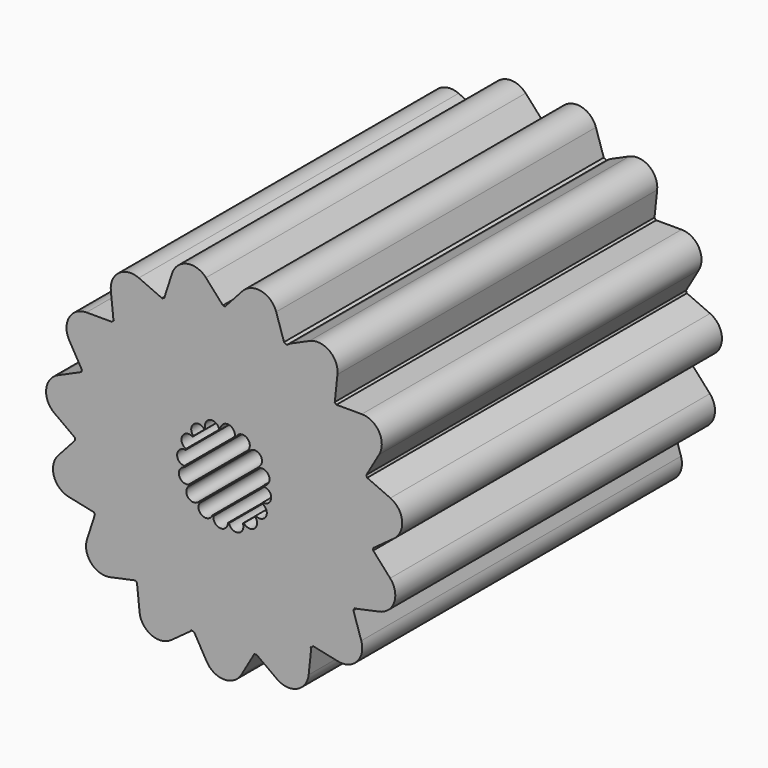
from build123d import *

# Parameters (mm, degrees)
F1_DEPTH    = 20
F2_T1_DEPTH = 28.6602540378
F2_T3_DEPTH = 21.427255965


# Not quite as in the source:
# - a fillet or chamfer that OpenCascade refuses, or shapes differently, is made with other operations: its cross-section is extruded or revolved along the edge and cut away or added


with BuildPart() as f1:
    # F0 (on Front) → F1 (new body)
    with BuildSketch(Plane.XZ):
        with BuildLine():
            Line((-32.6482919076, 40.6639489743), (-32.6758804008, 40.6333088485))
            ThreePointArc((-32.6758804008, 40.6333088485), (-33.545543461, 39.4533888073), (-34.6280952335, 38.4651546236))
            Line((-34.6280952335, 38.4651546236), (-34.6556837267, 38.4345144978))
            Line((-34.6556837267, 38.4345144978), (-31.7212409245, 37.8107794254))
            Line((-31.7212409245, 37.8107794254), (-32.6482919076, 40.6639489743))
        make_face()
        with BuildLine():
            Line((-37.6191296521, 37.1151033645), (-37.6603600082, 37.1151033645))
            ThreePointArc((-37.6603600082, 37.1151033645), (-39.1191296521, 36.971868355), (-40.5778992961, 37.1151033645))
            Line((-40.5778992961, 37.1151033645), (-40.6191296521, 37.1151033645))
            Line((-40.6191296521, 37.1151033645), (-39.1191296521, 34.5170271531))
            Line((-39.1191296521, 34.5170271531), (-37.6191296521, 37.1151033645))
        make_face()
        with BuildLine():
            Line((-40.7410773618, 37.1410241503), (-40.7787431663, 37.157794047))
            ThreePointArc((-40.7787431663, 37.157794047), (-42.1696544752, 37.6202774227), (-43.4440479302, 38.3444641829))
            Line((-43.4440479302, 38.3444641829), (-43.4817137347, 38.3612340796))
            Line((-43.4817137347, 38.3612340796), (-43.1681283449, 35.3776683935))
            Line((-43.1681283449, 35.3776683935), (-40.7410773618, 37.1410241503))
        make_face()
        with BuildLine():
            Line((-34.7565455695, 38.3612340796), (-34.794211374, 38.3444641829))
            ThreePointArc((-34.794211374, 38.3444641829), (-36.0686048291, 37.6202774227), (-37.4595161379, 37.157794047))
            Line((-37.4595161379, 37.157794047), (-37.4971819424, 37.1410241503))
            Line((-37.4971819424, 37.1410241503), (-35.0701309593, 35.3776683935))
            Line((-35.0701309593, 35.3776683935), (-34.7565455695, 38.3612340796))
        make_face()
        with BuildLine():
            Line((-43.5825755776, 38.4345144978), (-43.6101640707, 38.4651546236))
            ThreePointArc((-43.6101640707, 38.4651546236), (-44.6927158432, 39.4533888073), (-45.5623789035, 40.6333088485))
            Line((-45.5623789035, 40.6333088485), (-45.5899673966, 40.6639489743))
            Line((-45.5899673966, 40.6639489743), (-46.5170183798, 37.8107794254))
            Line((-46.5170183798, 37.8107794254), (-43.5825755776, 38.4345144978))
        make_face()
        with BuildLine():
            Line((-45.6523034437, 40.7719181749), (-45.6650443244, 40.8111305737))
            ThreePointArc((-45.6650443244, 40.8111305737), (-46.2520535243, 42.1542408972), (-46.5666135461, 43.5858753249))
            Line((-46.5666135461, 43.5858753249), (-46.5793544268, 43.6250877237))
            Line((-46.5793544268, 43.6250877237), (-48.5867462459, 41.3956532473))
            Line((-48.5867462459, 41.3956532473), (-45.6523034437, 40.7719181749))
        make_face()
        with BuildLine():
            ThreePointArc((-46.5880764634, 43.7900813429), (-46.5780438674, 45.2558318295), (-46.2831105651, 46.6916380453))
            Line((-46.2831105651, 46.6916380453), (-46.2788008194, 46.7326425371))
            Line((-46.2788008194, 46.7326425371), (-49.0194371923, 45.5124326079))
            Line((-49.0194371923, 45.5124326079), (-46.5923862092, 43.749076851))
            Line((-46.5923862092, 43.749076851), (-46.5880764634, 43.7900813429))
        make_face()
        with BuildLine():
            ThreePointArc((-46.2196598456, 46.8869192803), (-45.6143201805, 48.221868355), (-44.7608902016, 49.4135824202))
            Line((-44.7608902016, 49.4135824202), (-44.7402750236, 49.4492889559))
            Line((-44.7402750236, 49.4492889559), (-47.7402750236, 49.4492889559))
            Line((-47.7402750236, 49.4492889559), (-46.2402750236, 46.8512127446))
            Line((-46.2402750236, 46.8512127446), (-46.2196598456, 46.8869192803))
        make_face()
        with BuildLine():
            ThreePointArc((-44.623497051, 49.5661729728), (-43.5275190443, 50.5394958128), (-42.2631581853, 51.2810595392))
            Line((-42.2631581853, 51.2810595392), (-42.2298021266, 51.3052941344))
            Line((-42.2298021266, 51.3052941344), (-44.9704384995, 52.5255040636))
            Line((-44.9704384995, 52.5255040636), (-44.6568531097, 49.5419383775))
            Line((-44.6568531097, 49.5419383775), (-44.623497051, 49.5661729728))
        make_face()
        with BuildLine():
            ThreePointArc((-42.0755791275, 51.3645751165), (-40.6784673333, 51.8079753605), (-39.221795073, 51.9711656428))
            Line((-39.221795073, 51.9711656428), (-39.1814656992, 51.9797379159))
            Line((-39.1814656992, 51.9797379159), (-41.1888575182, 54.2091723923))
            Line((-41.1888575182, 54.2091723923), (-42.1159085014, 51.3560028434))
            Line((-42.1159085014, 51.3560028434), (-42.0755791275, 51.3645751165))
        make_face()
        with BuildLine():
            ThreePointArc((-39.0164642312, 51.9711656428), (-37.559791971, 51.8079753605), (-36.1626801768, 51.3645751165))
            Line((-36.1626801768, 51.3645751165), (-36.1223508029, 51.3560028434))
            Line((-36.1223508029, 51.3560028434), (-37.049401786, 54.2091723923))
            Line((-37.049401786, 54.2091723923), (-39.0567936051, 51.9797379159))
            Line((-39.0567936051, 51.9797379159), (-39.0164642312, 51.9711656428))
        make_face()
        with BuildLine():
            ThreePointArc((-35.9751011189, 51.2810595392), (-34.7107402599, 50.5394958128), (-33.6147622533, 49.5661729728))
            Line((-33.6147622533, 49.5661729728), (-33.5814061945, 49.5419383775))
            Line((-33.5814061945, 49.5419383775), (-33.2678208047, 52.5255040636))
            Line((-33.2678208047, 52.5255040636), (-36.0084571777, 51.3052941344))
            Line((-36.0084571777, 51.3052941344), (-35.9751011189, 51.2810595392))
        make_face()
        with BuildLine():
            ThreePointArc((-33.4773691026, 49.4135824202), (-32.6239391237, 48.221868355), (-32.0185994587, 46.8869192803))
            Line((-32.0185994587, 46.8869192803), (-31.9979842806, 46.8512127446))
            Line((-31.9979842806, 46.8512127446), (-30.4979842806, 49.4492889559))
            Line((-30.4979842806, 49.4492889559), (-33.4979842806, 49.4492889559))
            Line((-33.4979842806, 49.4492889559), (-33.4773691026, 49.4135824202))
        make_face()
        with BuildLine():
            ThreePointArc((-31.9551487391, 46.6916380453), (-31.7036102216, 45.5943974531), (-31.6191296521, 44.471868355))
            ThreePointArc((-31.6191296521, 44.471868355), (-31.6268969714, 44.1306214391), (-31.6501828408, 43.7900813429))
            Line((-31.6501828408, 43.7900813429), (-31.6458730951, 43.749076851))
            Line((-31.6458730951, 43.749076851), (-29.2188221119, 45.5124326079))
            Line((-29.2188221119, 45.5124326079), (-31.9594584849, 46.7326425371))
            Line((-31.9594584849, 46.7326425371), (-31.9551487391, 46.6916380453))
        make_face()
        with BuildLine():
            Line((-31.6589048775, 43.6250877237), (-31.6716457582, 43.5858753249))
            ThreePointArc((-31.6716457582, 43.5858753249), (-31.9862057799, 42.1542408972), (-32.5732149799, 40.8111305737))
            Line((-32.5732149799, 40.8111305737), (-32.5859558606, 40.7719181749))
            Line((-32.5859558606, 40.7719181749), (-29.6515130584, 41.3956532473))
            Line((-29.6515130584, 41.3956532473), (-31.6589048775, 43.6250877237))
        make_face()
        with BuildLine():
            ThreePointArc((-32.5732149799, 40.8111305737), (-31.9862057799, 42.1542408972), (-31.6716457582, 43.5858753249))
            Line((-31.6716457582, 43.5858753249), (-32.5732149799, 40.8111305737))
        make_face()
        with BuildLine():
            Line((-31.6501828408, 43.7900813429), (-31.9551487391, 46.6916380453))
            ThreePointArc((-31.9551487391, 46.6916380453), (-31.9862057799, 46.7894958128), (-32.0185994587, 46.8869192803))
            Line((-32.0185994587, 46.8869192803), (-33.4773691026, 49.4135824202))
            ThreePointArc((-33.4773691026, 49.4135824202), (-33.545543461, 49.4903479027), (-33.6147622533, 49.5661729728))
            Line((-33.6147622533, 49.5661729728), (-35.9751011189, 51.2810595392))
            ThreePointArc((-35.9751011189, 51.2810595392), (-36.0686048291, 51.3234592873), (-36.1626801768, 51.3645751165))
            Line((-36.1626801768, 51.3645751165), (-39.0164642312, 51.9711656428))
            ThreePointArc((-39.0164642312, 51.9711656428), (-39.1191296521, 51.971868355), (-39.221795073, 51.9711656428))
            Line((-39.221795073, 51.9711656428), (-42.0755791275, 51.3645751165))
            ThreePointArc((-42.0755791275, 51.3645751165), (-42.1696544752, 51.3234592873), (-42.2631581853, 51.2810595392))
            Line((-42.2631581853, 51.2810595392), (-44.623497051, 49.5661729728))
            ThreePointArc((-44.623497051, 49.5661729728), (-44.6927158432, 49.4903479027), (-44.7608902016, 49.4135824202))
            Line((-44.7608902016, 49.4135824202), (-46.2196598456, 46.8869192803))
            ThreePointArc((-46.2196598456, 46.8869192803), (-46.2520535243, 46.7894958128), (-46.2831105651, 46.6916380453))
            Line((-46.2831105651, 46.6916380453), (-46.5880764634, 43.7900813429))
            ThreePointArc((-46.5880764634, 43.7900813429), (-46.5780438674, 43.6879048805), (-46.5666135461, 43.5858753249))
            Line((-46.5666135461, 43.5858753249), (-45.6650443244, 40.8111305737))
            ThreePointArc((-45.6650443244, 40.8111305737), (-45.6143201805, 40.721868355), (-45.5623789035, 40.6333088485))
            Line((-45.5623789035, 40.6333088485), (-43.6101640707, 38.4651546236))
            ThreePointArc((-43.6101640707, 38.4651546236), (-43.5275190443, 38.4042408972), (-43.4440479302, 38.3444641829))
            Line((-43.4440479302, 38.3444641829), (-40.7787431663, 37.157794047))
            ThreePointArc((-40.7787431663, 37.157794047), (-40.6784673333, 37.1357613495), (-40.5778992961, 37.1151033645))
            Line((-40.5778992961, 37.1151033645), (-37.6603600082, 37.1151033645))
            ThreePointArc((-37.6603600082, 37.1151033645), (-37.559791971, 37.1357613495), (-37.4595161379, 37.157794047))
            Line((-37.4595161379, 37.157794047), (-34.794211374, 38.3444641829))
            ThreePointArc((-34.794211374, 38.3444641829), (-34.7107402599, 38.4042408972), (-34.6280952335, 38.4651546236))
            Line((-34.6280952335, 38.4651546236), (-32.6758804008, 40.6333088485))
            ThreePointArc((-32.6758804008, 40.6333088485), (-32.6239391237, 40.721868355), (-32.5732149799, 40.8111305737))
            Line((-32.5732149799, 40.8111305737), (-31.6716457582, 43.5858753249))
            ThreePointArc((-31.6716457582, 43.5858753249), (-31.6602154369, 43.6879048805), (-31.6501828408, 43.7900813429))
        make_face()
        with BuildLine():
            ThreePointArc((-37.1346171134, 44.7202832974), (-37.1310652132, 44.6900421087), (-37.1279741193, 44.6597503503))
            ThreePointArc((-37.1279741193, 44.6597503503), (-36.8713527385, 44.5542465364), (-36.7649469677, 44.2979978296))
            ThreePointArc((-36.7649469677, 44.2979978296), (-36.8945965479, 44.0205204586), (-37.1906148528, 43.9419337659))
            ThreePointArc((-37.1906148528, 43.9419337659), (-37.1989061268, 43.9126352973), (-37.2076424825, 43.8834664513))
            ThreePointArc((-37.2076424825, 43.8834664513), (-37.0444694696, 43.7502726214), (-36.9831488823, 43.5487637778))
            ThreePointArc((-36.9831488823, 43.5487637778), (-37.1713914481, 43.2313365827), (-37.5402114883, 43.2442619718))
            ThreePointArc((-37.5402114883, 43.2442619718), (-37.5590836652, 43.2203666495), (-37.5783174395, 43.1967614083))
            ThreePointArc((-37.5783174395, 43.1967614083), (-37.4992415442, 43.0790891384), (-37.4714606238, 42.9400640299))
            ThreePointArc((-37.4714606238, 42.9400640299), (-37.7249641514, 42.5948855598), (-38.1301841014, 42.7334821213))
            ThreePointArc((-38.1301841014, 42.7334821213), (-38.1567640633, 42.7186277915), (-38.1835670885, 42.704179839))
            ThreePointArc((-38.1835670885, 42.704179839), (-38.1626168369, 42.6357663211), (-38.155541156, 42.5645676047))
            ThreePointArc((-38.155541156, 42.5645676047), (-38.4784656795, 42.2049028746), (-38.8707147097, 42.4873558163))
            ThreePointArc((-38.8707147097, 42.4873558163), (-38.9009558984, 42.4838039161), (-38.9312476568, 42.4807128222))
            ThreePointArc((-38.9312476568, 42.4807128222), (-38.9312459786, 42.4800766266), (-38.9312454191, 42.479440429))
            ThreePointArc((-38.9312454191, 42.479440429), (-39.3250831627, 42.1191111528), (-39.6490642412, 42.5433535556))
            ThreePointArc((-39.6490642412, 42.5433535556), (-39.6783627098, 42.5516448297), (-39.7075315558, 42.5603811853))
            ThreePointArc((-39.7075315558, 42.5603811853), (-40.2092029659, 42.3767249926), (-40.3467360353, 42.8929501912))
            ThreePointArc((-40.3467360353, 42.8929501912), (-40.3706313576, 42.9118223681), (-40.3942365988, 42.9310561424))
            ThreePointArc((-40.3942365988, 42.9310561424), (-40.9280027289, 42.953361282), (-40.8575158859, 43.4829228043))
            ThreePointArc((-40.8575158859, 43.4829228043), (-40.8723702156, 43.5095027662), (-40.8868181681, 43.5363057913))
            ThreePointArc((-40.8868181681, 43.5363057913), (-41.3714179634, 43.761176508), (-41.1036421909, 44.2234534126))
            ThreePointArc((-41.1036421909, 44.2234534126), (-41.107194091, 44.2536946013), (-41.1102851849, 44.2839863597))
            ThreePointArc((-41.1102851849, 44.2839863597), (-41.4719427196, 44.6771881253), (-41.0476444515, 45.001802944))
            ThreePointArc((-41.0476444515, 45.001802944), (-41.0393531774, 45.0311014127), (-41.0306168218, 45.0602702587))
            ThreePointArc((-41.0306168218, 45.0602702587), (-41.2142730146, 45.5619416688), (-40.6980478159, 45.6994747382))
            ThreePointArc((-40.6980478159, 45.6994747382), (-40.679175639, 45.7233700605), (-40.6599418647, 45.7469753017))
            ThreePointArc((-40.6599418647, 45.7469753017), (-40.6376367251, 46.2807414318), (-40.1080752029, 46.2102545887))
            ThreePointArc((-40.1080752029, 46.2102545887), (-40.0814952409, 46.2251089185), (-40.0546922158, 46.239556871))
            ThreePointArc((-40.0546922158, 46.239556871), (-39.8298214991, 46.7241566663), (-39.3675445945, 46.4563808937))
            ThreePointArc((-39.3675445945, 46.4563808937), (-39.3373034058, 46.4599327939), (-39.3070116474, 46.4630238878))
            ThreePointArc((-39.3070116474, 46.4630238878), (-38.9458953243, 46.82605048), (-38.5835043684, 46.464296281))
            ThreePointArc((-38.5835043684, 46.464296281), (-38.5849298506, 46.4322132958), (-38.5891950631, 46.4003831543))
            ThreePointArc((-38.5891950631, 46.4003831543), (-38.5598965945, 46.3920918803), (-38.5307277484, 46.3833555246))
            ThreePointArc((-38.5307277484, 46.3833555246), (-38.126074305, 46.6010216758), (-37.8342703166, 46.2460943664))
            ThreePointArc((-37.8342703166, 46.2460943664), (-37.8488785047, 46.1443310922), (-37.8915232689, 46.0507865188))
            ThreePointArc((-37.8915232689, 46.0507865188), (-37.8676279467, 46.0319143419), (-37.8440227054, 46.0126805676))
            ThreePointArc((-37.8440227054, 46.0126805676), (-37.4494757585, 46.0922433874), (-37.2255705687, 45.757782625))
            ThreePointArc((-37.2255705687, 45.757782625), (-37.2667021108, 45.5902497674), (-37.3807434184, 45.4608139057))
            ThreePointArc((-37.3807434184, 45.4608139057), (-37.3658890886, 45.4342339438), (-37.3514411361, 45.4074309186))
            ThreePointArc((-37.3514411361, 45.4074309186), (-37.0113780162, 45.3748431687), (-36.8500741435, 45.0737020928))
            ThreePointArc((-36.8500741435, 45.0737020928), (-36.9300504099, 44.8468378455), (-37.1346171134, 44.7202832974))
        make_face(mode=Mode.SUBTRACT)
        with BuildLine():
            ThreePointArc((-46.5666135461, 43.5858753249), (-46.2520535243, 42.1542408972), (-45.6650443244, 40.8111305737))
            Line((-45.6650443244, 40.8111305737), (-46.5666135461, 43.5858753249))
        make_face()
        with BuildLine():
            Line((-35.9751011189, 51.2810595392), (-33.6147622533, 49.5661729728))
            ThreePointArc((-33.6147622533, 49.5661729728), (-34.7107402599, 50.5394958128), (-35.9751011189, 51.2810595392))
        make_face()
        with BuildLine():
            Line((-39.0164642312, 51.9711656428), (-36.1626801768, 51.3645751165))
            ThreePointArc((-36.1626801768, 51.3645751165), (-37.559791971, 51.8079753605), (-39.0164642312, 51.9711656428))
        make_face()
        with BuildLine():
            ThreePointArc((-45.5623789035, 40.6333088485), (-44.6927158432, 39.4533888073), (-43.6101640707, 38.4651546236))
            Line((-43.6101640707, 38.4651546236), (-45.5623789035, 40.6333088485))
        make_face()
        with BuildLine():
            Line((-33.4773691026, 49.4135824202), (-32.0185994587, 46.8869192803))
            ThreePointArc((-32.0185994587, 46.8869192803), (-32.6239391237, 48.221868355), (-33.4773691026, 49.4135824202))
        make_face()
        with BuildLine():
            Line((-46.5880764634, 43.7900813429), (-46.2831105651, 46.6916380453))
            ThreePointArc((-46.2831105651, 46.6916380453), (-46.5780438674, 45.2558318295), (-46.5880764634, 43.7900813429))
        make_face()
        with BuildLine():
            ThreePointArc((-34.6280952335, 38.4651546236), (-33.545543461, 39.4533888073), (-32.6758804008, 40.6333088485))
            Line((-32.6758804008, 40.6333088485), (-34.6280952335, 38.4651546236))
        make_face()
        with BuildLine():
            ThreePointArc((-31.6501828408, 43.7900813429), (-31.6268969714, 44.1306214391), (-31.6191296521, 44.471868355))
            ThreePointArc((-31.6191296521, 44.471868355), (-31.7036102216, 45.5943974531), (-31.9551487391, 46.6916380453))
            Line((-31.9551487391, 46.6916380453), (-31.6501828408, 43.7900813429))
        make_face()
        with BuildLine():
            ThreePointArc((-40.5778992961, 37.1151033645), (-39.1191296521, 36.971868355), (-37.6603600082, 37.1151033645))
            Line((-37.6603600082, 37.1151033645), (-40.5778992961, 37.1151033645))
        make_face()
        with BuildLine():
            Line((-44.623497051, 49.5661729728), (-42.2631581853, 51.2810595392))
            ThreePointArc((-42.2631581853, 51.2810595392), (-43.5275190443, 50.5394958128), (-44.623497051, 49.5661729728))
        make_face()
        with BuildLine():
            Line((-42.0755791275, 51.3645751165), (-39.221795073, 51.9711656428))
            ThreePointArc((-39.221795073, 51.9711656428), (-40.6784673333, 51.8079753605), (-42.0755791275, 51.3645751165))
        make_face()
        with BuildLine():
            Line((-46.2196598456, 46.8869192803), (-44.7608902016, 49.4135824202))
            ThreePointArc((-44.7608902016, 49.4135824202), (-45.6143201805, 48.221868355), (-46.2196598456, 46.8869192803))
        make_face()
        with BuildLine():
            ThreePointArc((-37.4595161379, 37.157794047), (-36.0686048291, 37.6202774227), (-34.794211374, 38.3444641829))
            Line((-34.794211374, 38.3444641829), (-37.4595161379, 37.157794047))
        make_face()
        with BuildLine():
            ThreePointArc((-43.4440479302, 38.3444641829), (-42.1696544752, 37.6202774227), (-40.7787431663, 37.157794047))
            Line((-40.7787431663, 37.157794047), (-43.4440479302, 38.3444641829))
        make_face()
    extrude(amount=F1_DEPTH)

    # F2: fillet of radius 1 on 16 edges, made by hand

    # F2_s2 → F2_t1 (cut)
    with BuildSketch(Plane.XZ.offset(-4.3301270189)):
        with BuildLine():
            ThreePointArc((-31.3640096844, 47.9492889559), (-31.3640096844, 48.9492889559), (-32.2300350882, 49.4492889559))
            Line((-32.2300350882, 49.4492889559), (-30.4979842806, 49.4492889559))
            Line((-30.4979842806, 49.4492889559), (-31.3640096844, 47.9492889559))
        make_face()
        with BuildLine():
            ThreePointArc((-30.6200806504, 44.494358687), (-30.2133440073, 45.4079041446), (-30.8011292596, 46.216921139))
            Line((-30.8011292596, 46.216921139), (-29.2188221119, 45.5124326079))
            Line((-29.2188221119, 45.5124326079), (-30.6200806504, 44.494358687))
        make_face()
        with BuildLine():
            ThreePointArc((-31.3457144002, 41.0355396353), (-30.6025695747, 41.7046702417), (-30.8104812655, 42.6828178424))
            Line((-30.8104812655, 42.6828178424), (-29.6515130584, 41.3956532473))
            Line((-29.6515130584, 41.3956532473), (-31.3457144002, 41.0355396353))
        make_face()
        with BuildLine():
            ThreePointArc((-33.4154422663, 38.1708930374), (-32.46438575, 38.4799100317), (-32.2564740592, 39.4580576325))
            Line((-32.2564740592, 39.4580576325), (-31.7212409245, 37.8107794254))
            Line((-31.7212409245, 37.8107794254), (-33.4154422663, 38.1708930374))
        make_face()
        with BuildLine():
            ThreePointArc((-36.4713894978, 36.3957423144), (-35.4768676024, 36.2912138511), (-34.8890823501, 37.1002308455))
            Line((-34.8890823501, 37.1002308455), (-35.0701309593, 35.3776683935))
            Line((-35.0701309593, 35.3776683935), (-36.4713894978, 36.3957423144))
        make_face()
        with BuildLine():
            ThreePointArc((-39.9851550559, 36.0170271531), (-39.1191296521, 35.5170271531), (-38.2531042483, 36.0170271531))
            Line((-38.2531042483, 36.0170271531), (-39.1191296521, 34.5170271531))
            Line((-39.1191296521, 34.5170271531), (-39.9851550559, 36.0170271531))
        make_face()
        with BuildLine():
            ThreePointArc((-43.3491769541, 37.1002308455), (-42.7613917019, 36.2912138511), (-41.7668698065, 36.3957423144))
            Line((-41.7668698065, 36.3957423144), (-43.1681283449, 35.3776683935))
            Line((-43.1681283449, 35.3776683935), (-43.3491769541, 37.1002308455))
        make_face()
        with BuildLine():
            ThreePointArc((-45.9817852451, 39.4580576325), (-45.7738735543, 38.4799100317), (-44.822817038, 38.1708930374))
            Line((-44.822817038, 38.1708930374), (-46.5170183798, 37.8107794254))
            Line((-46.5170183798, 37.8107794254), (-45.9817852451, 39.4580576325))
        make_face()
        with BuildLine():
            ThreePointArc((-33.448869414, 50.8029416116), (-33.855606057, 51.7164870692), (-34.8501279524, 51.8210155325))
            Line((-34.8501279524, 51.8210155325), (-33.2678208047, 52.5255040636))
            Line((-33.2678208047, 52.5255040636), (-33.448869414, 50.8029416116))
        make_face()
        with BuildLine():
            ThreePointArc((-40.0298893111, 52.9220077972), (-40.9809458274, 53.2310247916), (-41.7240906529, 52.5618941852))
            Line((-41.7240906529, 52.5618941852), (-41.1888575182, 54.2091723923))
            Line((-41.1888575182, 54.2091723923), (-40.0298893111, 52.9220077972))
        make_face()
        with BuildLine():
            ThreePointArc((-43.3881313518, 51.8210155325), (-44.3826532472, 51.7164870692), (-44.7893898903, 50.8029416116))
            Line((-44.7893898903, 50.8029416116), (-44.9704384995, 52.5255040636))
            Line((-44.9704384995, 52.5255040636), (-43.3881313518, 51.8210155325))
        make_face()
        with BuildLine():
            ThreePointArc((-46.008224216, 49.4492889559), (-46.8742496198, 48.9492889559), (-46.8742496198, 47.9492889559))
            Line((-46.8742496198, 47.9492889559), (-47.7402750236, 49.4492889559))
            Line((-47.7402750236, 49.4492889559), (-46.008224216, 49.4492889559))
        make_face()
        with BuildLine():
            ThreePointArc((-47.4371300447, 46.216921139), (-48.0249152969, 45.4079041446), (-47.6181786539, 44.494358687))
            Line((-47.6181786539, 44.494358687), (-49.0194371923, 45.5124326079))
            Line((-49.0194371923, 45.5124326079), (-47.4371300447, 46.216921139))
        make_face()
        with BuildLine():
            ThreePointArc((-47.4277780387, 42.6828178424), (-47.6356897296, 41.7046702417), (-46.8925449041, 41.0355396353))
            Line((-46.8925449041, 41.0355396353), (-48.5867462459, 41.3956532473))
            Line((-48.5867462459, 41.3956532473), (-47.4277780387, 42.6828178424))
        make_face()
        with BuildLine():
            ThreePointArc((-36.5141686514, 52.5618941852), (-37.2573134768, 53.2310247916), (-38.2083699931, 52.9220077972))
            Line((-38.2083699931, 52.9220077972), (-37.049401786, 54.2091723923))
            Line((-37.049401786, 54.2091723923), (-36.5141686514, 52.5618941852))
        make_face()
    extrude(amount=F2_T1_DEPTH, mode=Mode.SUBTRACT)

    # F2_s4 → F2_t3 (cut)
    with BuildSketch(Plane.XZ.offset(-0.7136279825)):
        with BuildLine():
            ThreePointArc((-35.7476845369, 51.4213975944), (-35.8661017968, 51.3588594094), (-35.9751011189, 51.2810595392))
            Line((-35.9751011189, 51.2810595392), (-36.0084571777, 51.3052941344))
            Line((-36.0084571777, 51.3052941344), (-35.7476845369, 51.4213975944))
        make_face()
    extrude(amount=F2_T3_DEPTH, mode=Mode.SUBTRACT)


solid = f1.part
